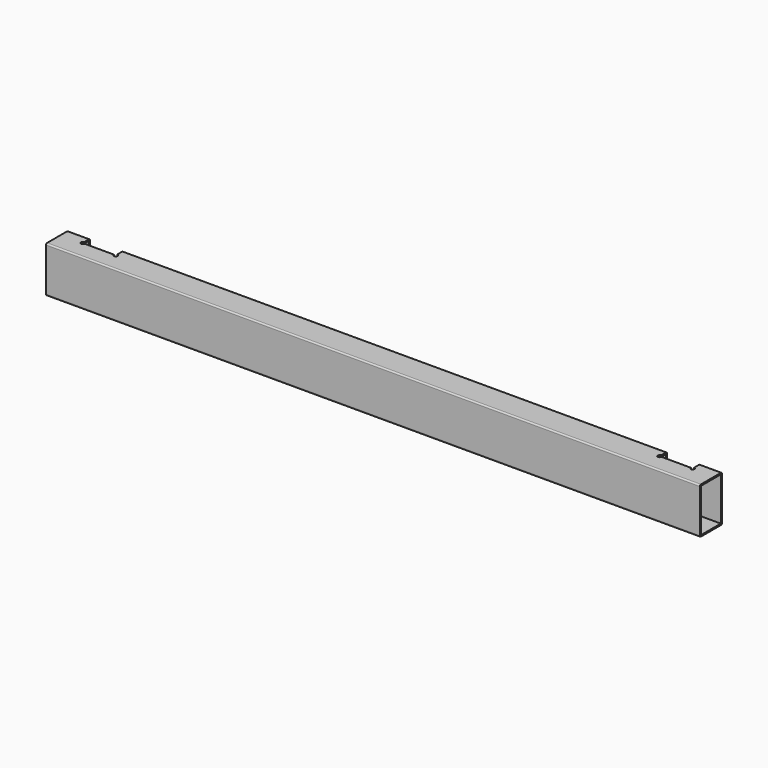
from build123d import *

# Parameters (mm, degrees)
F0_W     = 54
F0_H     = 94
F1_DEPTH = 710
F3_START = 20
F3_DEPTH = 35
F4_START = 20
F4_DEPTH = 35


with BuildPart() as f1:
    # F0 (on Right) → F1 (new body, symmetric)
    with BuildSketch(Plane.YZ):
        with BuildLine():
            ThreePointArc((30, 47), (29.1213203436, 49.1213203436), (27, 50))
            Line((27, 50), (-27, 50))
            ThreePointArc((-27, 50), (-29.1213203436, 49.1213203436), (-30, 47))
            Line((-30, 47), (-30, -47))
            ThreePointArc((-30, -47), (-29.1213203436, -49.1213203436), (-27, -50))
            Line((-27, -50), (27, -50))
            ThreePointArc((27, -50), (29.1213203436, -49.1213203436), (30, -47))
            Line((30, -47), (30, 47))
        make_face()
        Rectangle(F0_W, F0_H, mode=Mode.SUBTRACT)
    extrude(amount=F1_DEPTH, both=True)

    # F2 (on Top) → F3 (cut)
    with BuildSketch(Plane.XY.offset(F3_START)):
        with BuildLine():
            Line((-590.61, 40), (-662.61, 40))
            Line((-662.61, 40), (-662.61, 14))
            ThreePointArc((-662.61, 14), (-665.4384271247, 7.1715728753), (-658.61, 10))
            Line((-658.61, 10), (-594.61, 10))
            ThreePointArc((-594.61, 10), (-587.7815728753, 7.1715728753), (-590.61, 14))
            Line((-590.61, 14), (-590.61, 40))
        make_face()
    extrude(amount=F3_DEPTH, mode=Mode.SUBTRACT)

    # F2 (on Top) → F4 (cut)
    with BuildSketch(Plane.XY.offset(F4_START)):
        with BuildLine():
            Line((662.61, 14), (662.61, 40))
            Line((662.61, 40), (590.61, 40))
            Line((590.61, 40), (590.61, 14))
            ThreePointArc((590.61, 14), (587.7815728753, 7.1715728753), (594.61, 10))
            Line((594.61, 10), (658.61, 10))
            ThreePointArc((658.61, 10), (665.4384271247, 7.1715728753), (662.61, 14))
        make_face()
    extrude(amount=F4_DEPTH, mode=Mode.SUBTRACT)


solid = f1.part
